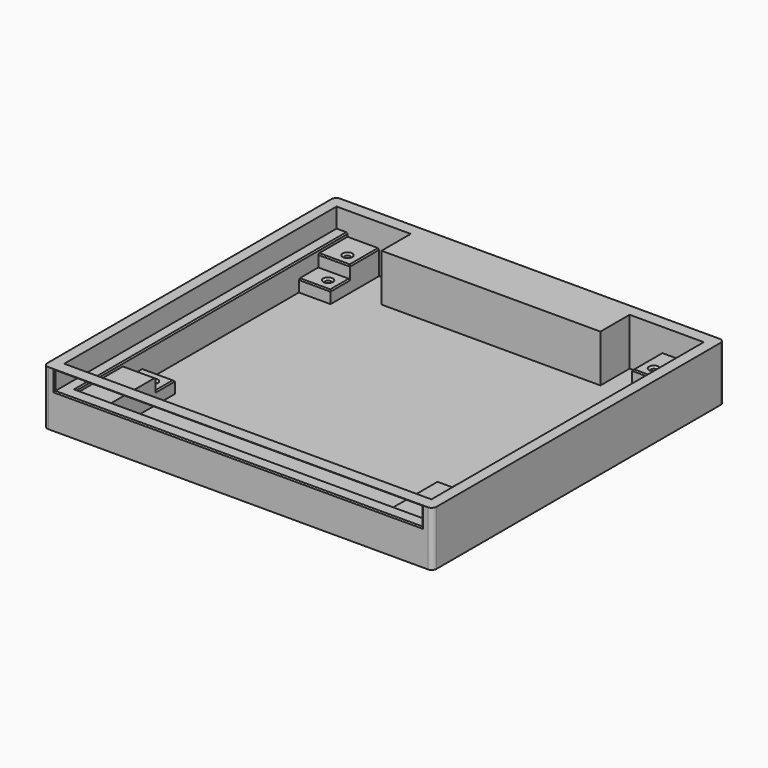
from build123d import *

# Parameters (mm, degrees)
F1_DEPTH             = 3
F2_W                 = 10
F2_H                 = 10
F3_DEPTH             = 5
F5_W                 = 10
F5_H                 = 10
F6_DEPTH             = 10
F8_D                 = 2.5
F8_DEPTH             = 5
F8_CSINK_D           = 4
F8_CSINK_ANGLE       = 90
F8_TIP               = 0.7510757738
F8_ON_F4_D           = 2.5
F8_ON_F4_DEPTH       = 5
F8_ON_F4_CSINK_D     = 4
F8_ON_F4_CSINK_ANGLE = 90
F8_ON_F4_TIP         = 0.7510757738
F9_W                 = 9
F9_H                 = 140
F10_DEPTH            = 11.5
F11_W                = 4.5
F11_H                = 140
F12_DEPTH            = 8
F14_DEPTH            = 19.5
F15_W                = 151
F15_H                = 7.5
F16_DEPTH            = 5
F18_DEPTH            = 3
F19_W                = 13
F19_H                = 10
F19_W_2              = 10
F20_DEPTH            = 5
F22_DEPTH            = 3
F23_W                = 13
F23_H                = 10
F24_DEPTH            = 15
F25_W                = 90
F25_H                = 15
F26_DEPTH            = 19.5
F27_SIZE             = 0.49999


# Not quite as in the source:
# - a fillet or chamfer is up to 0.001 mm smaller than in the source, because OpenCascade refuses the exact size
# - a feature names something its author has since deleted; it is built from what else it names


with BuildPart() as f1:
    # F0 (on Top) → F1 (new body)
    with BuildSketch(Plane.XY):
        with BuildLine():
            Line((-78, -75), (78, -75))
            ThreePointArc((78, -75), (79.4142135624, -74.4142135624), (80, -73))
            Line((80, -73), (80, 73))
            ThreePointArc((80, 73), (79.4142135624, 74.4142135624), (78, 75))
            Line((78, 75), (-78, 75))
            ThreePointArc((-78, 75), (-79.4142135624, 74.4142135624), (-80, 73))
            Line((-80, 73), (-80, -73))
            ThreePointArc((-80, -73), (-79.4142135624, -74.4142135624), (-78, -75))
        make_face()
    extrude(amount=F1_DEPTH)

    # F2 (on face) → F3 (join)
    with BuildSketch(Plane.XY.offset(3)):
        with Locations((-63, -40)):
            Rectangle(F2_W, F2_H)
        with Locations((-63, 50)):
            Rectangle(F2_W, F2_H)
        with Locations((63, 50)):
            Rectangle(F2_W, F2_H)
        with Locations((63, -40)):
            Rectangle(F2_W, F2_H)
    extrude(amount=F3_DEPTH)

    # F5 (on face) → F6 (join)
    with BuildSketch(Plane.XY.offset(3)):
        with Locations((-63, 60)):
            Rectangle(F5_W, F5_H)
        with Locations((-63, -50)):
            Rectangle(F5_W, F5_H)
        with Locations((63, 60)):
            Rectangle(F5_W, F5_H)
        with Locations((63, -50)):
            Rectangle(F5_W, F5_H)
    extrude(amount=F6_DEPTH)

    # F8
    with Locations(Plane.XY.offset(13)):
        with Locations((-63, 60), (63, 60)):
            CounterSinkHole(F8_D / 2, F8_CSINK_D / 2, depth=F8_DEPTH, counter_sink_angle=F8_CSINK_ANGLE)
            with Locations((0, 0, -(F8_DEPTH + F8_TIP / 2))):  # 118° drill point
                Cone(0, F8_D / 2, F8_TIP, mode=Mode.SUBTRACT)

    # F8 on F4
    with Locations(Plane.XY.offset(8)):
        with Locations((-63, -40), (63, -40), (-63, 50), (63, 50)):
            CounterSinkHole(F8_ON_F4_D / 2, F8_ON_F4_CSINK_D / 2, depth=F8_ON_F4_DEPTH, counter_sink_angle=F8_ON_F4_CSINK_ANGLE)
            with Locations((0, 0, -(F8_ON_F4_DEPTH + F8_ON_F4_TIP / 2))):  # 118° drill point
                Cone(0, F8_ON_F4_D / 2, F8_ON_F4_TIP, mode=Mode.SUBTRACT)

    # F9 (on face) → F10 (join)
    with BuildSketch(Plane.XY.offset(3)):
        with Locations((-75.5, 0)):
            Rectangle(F9_W, F9_H)
        with Locations((75.5, 0)):
            Rectangle(F9_W, F9_H)
    extrude(amount=F10_DEPTH)

    # F11 (on face) → F12 (join)
    with BuildSketch(Plane.XY.offset(14.5)):
        with Locations((-77.75, 0)):
            Rectangle(F11_W, F11_H)
        with Locations((77.75, 0)):
            Rectangle(F11_W, F11_H)
    extrude(amount=F12_DEPTH)

    # F13 (on face) → F14 (join, through all)
    with BuildSketch(Plane.XY.offset(3)):
        with BuildLine():
            Line((-80, -70), (-80, -73))
            ThreePointArc((-80, -73), (-79.4142135624, -74.4142135624), (-78, -75))
            Line((-78, -75), (78, -75))
            ThreePointArc((78, -75), (79.4142135624, -74.4142135624), (80, -73))
            Line((80, -73), (80, -70))
            Line((80, -70), (-80, -70))
        make_face()
        with BuildLine():
            Line((-80, 73), (-80, 70))
            Line((-80, 70), (80, 70))
            Line((80, 70), (80, 73))
            ThreePointArc((80, 73), (79.4142135624, 74.4142135624), (78, 75))
            Line((78, 75), (-78, 75))
            ThreePointArc((-78, 75), (-79.4142135624, 74.4142135624), (-80, 73))
        make_face()
    extrude(amount=F14_DEPTH)

    # F15 (on face) → F16 (cut, through all)
    with BuildSketch(Plane.XZ.offset(75)):
        with Locations((0, 18.25)):
            Rectangle(F15_W, F15_H)
    extrude(amount=-F16_DEPTH, mode=Mode.SUBTRACT)

    # F17 (on face) → F18 (join, through all)
    with BuildSketch(Plane(origin=(-68, 0, 0), x_dir=(0, -1, 0), z_dir=(-1, 0, 0))):
        Polygon((-65, 3), (-45, 3), (-45, 8), (-55, 8), (-55, 13), (-65, 13), align=None)
        Polygon((35, 3), (55, 3), (55, 13), (45, 13), (45, 8), (35, 8), align=None)
    extrude(amount=F18_DEPTH)

    # F19 (on face) → F20 (join, through all)
    with BuildSketch(Plane(origin=(0, 65, 0), x_dir=(-1, 0, 0), z_dir=(0, 1, 0))):
        with Locations((64.5, 8)):
            Rectangle(F19_W, F19_H)
        with Locations((-63, 8)):
            Rectangle(F19_W_2, F19_H)
    extrude(amount=F20_DEPTH)

    # F21 (on face) → F22 (join, through all)
    with BuildSketch(Plane.YZ.offset(68)):
        Polygon((45, 8), (45, 3), (70, 3), (70, 13), (55, 13), (55, 8), align=None)
        Polygon((-55, 13), (-55, 3), (-35, 3), (-35, 8), (-45, 8), (-45, 13), align=None)
    extrude(amount=F22_DEPTH)

    # F23 (on face) → F24 (join, through all)
    with BuildSketch(Plane.XZ.offset(55)):
        with Locations((64.5, 8)):
            Rectangle(F23_W, F23_H)
        with Locations((-64.5, 8)):
            Rectangle(F23_W, F23_H)
    extrude(amount=F24_DEPTH)

    # F25 (on face) → F26 (join, through all)
    with BuildSketch(Plane.XY.offset(3)):
        with Locations((0, 62.5)):
            Rectangle(F25_W, F25_H)
    extrude(amount=F26_DEPTH)

    # F27 (size 0.5 in the source; OpenCascade refuses exactly that, so slightly less here)
    f27_edges = [f1.edges().sort_by_distance(p)[0] for p in [
        (71, 0, 14.5),
        (-71, 0, 14.5),
        (-58, 62.5, 13),
        (-64.5, 55, 13),
        (-58, 50, 8),
        (-64.5, 45, 8),
        (-64.5, -45, 13),
        (-58, -40, 8),
        (-64.5, -35, 8),
        (58, 62.5, 13),
        (64.5, 55, 13),
        (58, 50, 8),
        (64.5, 45, 8),
        (-75.5, -75, 18.25),
        (0, -75, 14.5),
        (0, -75, 22),
        (75.5, -75, 18.25),
    ]]
    chamfer(f27_edges, length=F27_SIZE)


solid = f1.part
